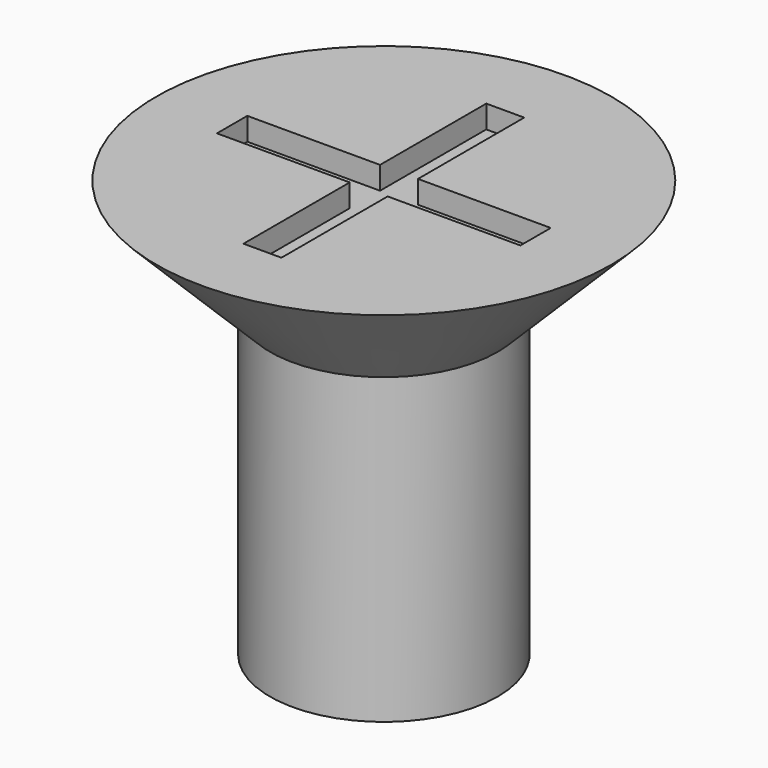
from build123d import *

# Parameters (mm, degrees)
F0_R     = 3
F1_DEPTH = 1.5
F2_SIZE  = 1.49999
F3_W     = 0.5
F3_H     = 1.75
F3_H_2   = 0.5
F3_W_2   = 1.75
F4_DEPTH = 0.3
F5_DEPTH = 4


# Not quite as in the source:
# - a fillet or chamfer is up to 0.001 mm smaller than in the source, because OpenCascade refuses the exact size


with BuildPart() as f1:
    # F0 (on Top) → F1 (new body)
    with BuildSketch(Plane.XY):
        with Locations((3.0322743114, 7.5806910172)):
            Circle(F0_R)
    extrude(amount=F1_DEPTH)

    # F2 (size 1.5 in the source; OpenCascade refuses exactly that, so slightly less here)
    f2_edges = [f1.edges().sort_by_distance(p)[0] for p in [
        (0.032274, 7.580691, 0),
    ]]
    chamfer(f2_edges, length=F2_SIZE)

    # F3 (on face) → F4 (cut)
    with BuildSketch(Plane.XY.offset(1.5)):
        with Locations((3.0322743114, 8.7056910172)):
            Rectangle(F3_W, F3_H)
        with Locations((3.0322743114, 7.5806910172)):
            Rectangle(F3_W, F3_H_2)
        with Locations((1.9072743114, 7.5806910172)):
            Rectangle(F3_W_2, F3_H_2)
        with Locations((4.1572743114, 7.5806910172)):
            Rectangle(F3_W_2, F3_H_2)
        Polygon((3.2822743114, 7.3306910172), (2.7822743114, 7.3306910172), (2.7822743114, 5.5806910172), (3.0322743114, 5.5806910172), (3.2822743114, 5.5806910172), align=None)
    extrude(amount=-F4_DEPTH, mode=Mode.SUBTRACT)

    # F5 (add): a face of the model
    f5_faces = [f1.faces().sort_by_distance(p)[0] for p in [
        (3.0322743114, 7.5806910172, 0),
    ]]
    extrude(f5_faces, amount=F5_DEPTH)


solid = f1.part
